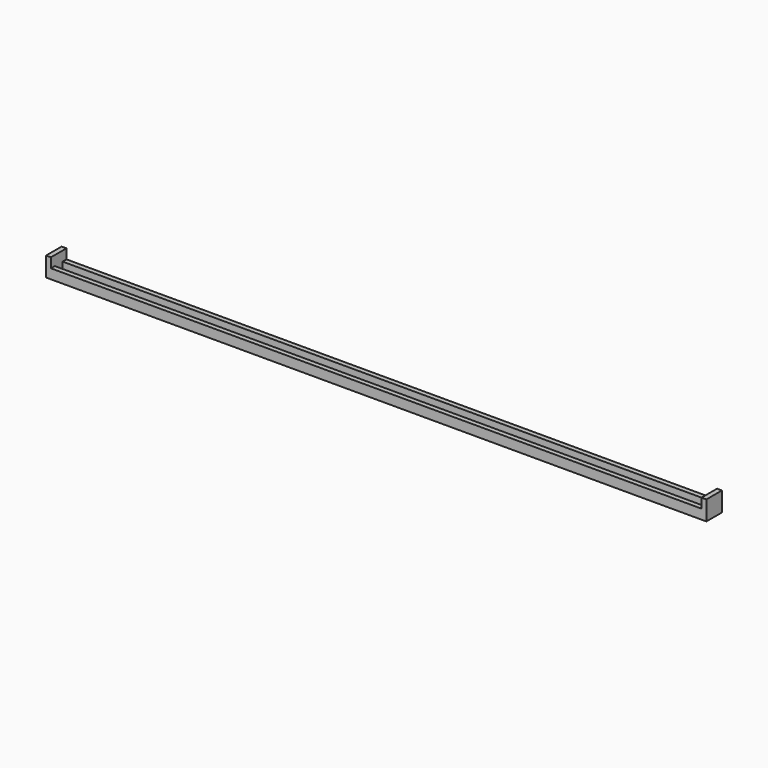
from build123d import *

# Parameters (mm, degrees)
F0_W     = 215.9
F0_H     = 6.35
F0_W_2   = 212.725
F0_H_2   = 3.175
F1_DEPTH = 3.175
F3_DEPTH = 3.175


# Not quite as in the source:
# - a length typed as a fraction of an inch, garbled in the dataset ("3 / 203.2 mm" for 3/8 in), is restored


with BuildPart() as f1:
    # F0 (on Top) → F1 (new body)
    with BuildSketch(Plane.XY):
        with Locations((107.95, 3.175)):
            Rectangle(F0_W, F0_H)
        with Locations((107.95, 3.175)):
            Rectangle(F0_W_2, F0_H_2, mode=Mode.SUBTRACT)
    extrude(amount=F1_DEPTH)

    # F2 (on face) → F3 (join)
    with BuildSketch(Plane.XY.offset(3.175)):
        Polygon((1.5875, 0), (1.5875, 1.5875), (1.5875, 4.7625), (1.5875, 6.35), (0, 6.35), (0, 0), align=None)
        Polygon((214.3125, 4.7625), (214.3125, 1.5875), (214.3125, 0), (215.9, 0), (215.9, 6.35), (214.3125, 6.35), align=None)
    extrude(amount=F3_DEPTH)


solid = f1.part
